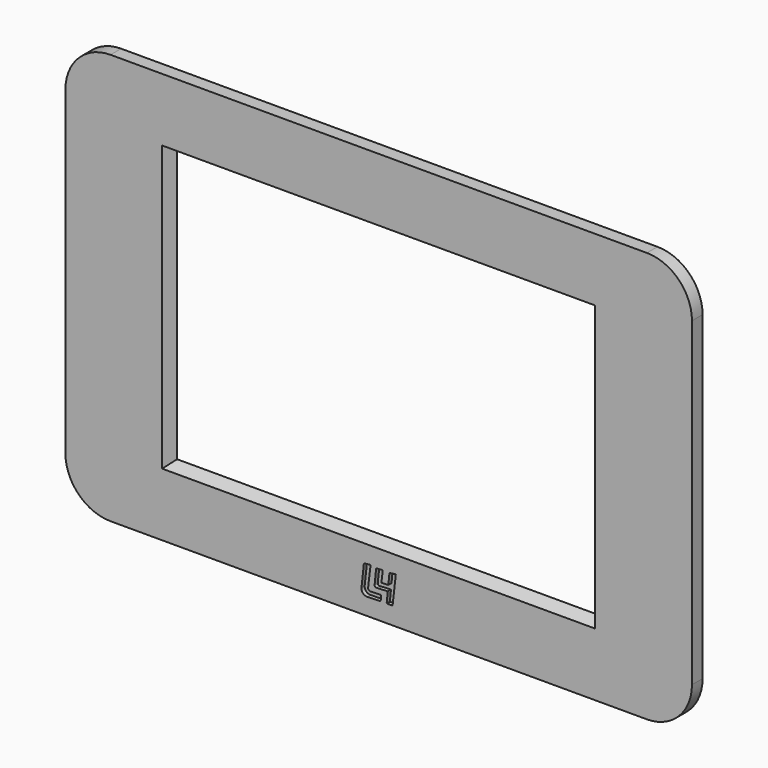
from build123d import *

# Parameters (mm, degrees)
F0_W     = 236.2
F0_H     = 154.8
F0_W_2   = 160
F0_H_2   = 104
F1_DEPTH = 5
F2_R     = 17
F3_R     = 3.25
F4_DEPTH = 2.5
F5_SIZE2 = 4.99999
F5_SIZE  = 1.624588
F7_DEPTH = 1.5


# Not quite as in the source:
# - a fillet or chamfer is up to 0.001 mm smaller than in the source, because OpenCascade refuses the exact size


with BuildPart() as f1:
    # F0 (on Front) → F1 (new body)
    with BuildSketch(Plane.XZ):
        Rectangle(F0_W, F0_H)
        Rectangle(F0_W_2, F0_H_2, mode=Mode.SUBTRACT)
    extrude(amount=F1_DEPTH)

    # F2
    f2_edges = [f1.edges().sort_by_distance(p)[0] for p in [
        (-118.1, -2.5, 77.4),
        (118.1, -2.5, 77.4),
        (-118.1, -2.5, -77.4),
        (118.1, -2.5, -77.4),
    ]]
    fillet(f2_edges, radius=F2_R)

    # F3 (on face) → F4 (cut)
    with BuildSketch(Plane(origin=(0, 0, 0), x_dir=(-1, 0, 0), z_dir=(0, 1, 0))):
        with Locations((-79.25, 66.42428)):
            Circle(F3_R)
        with Locations((-79.25, -66.42428)):
            Circle(F3_R)
        with Locations((79.25, 66.42428)):
            Circle(F3_R)
        with Locations((79.25, -66.42428)):
            Circle(F3_R)
    extrude(amount=-F4_DEPTH, mode=Mode.SUBTRACT)

    # F5 (size 1.6245984812 and 5 in the source; OpenCascade refuses exactly that, so slightly less here)
    f5_edges = [f1.edges().sort_by_distance(p)[0] for p in [
        (-80, -5, 0),
        (0, -5, 52),
        (80, -5, 0),
        (0, -5, -52),
    ]]
    f5_side = f1.faces().sort_by_distance((0, -5, 74.575934))[0]
    chamfer(f5_edges, length=F5_SIZE, length2=F5_SIZE2, reference=f5_side)

    # F6 (on face) → F7 (cut)
    with BuildSketch(Plane.XZ.offset(5)):
        with BuildLine():
            Line((0, -70.9037960887), (0, -68.7403732376))
            Line((0, -68.7403732376), (-3.125376912, -68.8479899255))
            ThreePointArc((-3.125376912, -68.8479899255), (-3.7805726372, -68.5735525412), (-3.998605605, -67.897491197))
            Line((-3.998605605, -67.897491197), (-3.0892937711, -60.2992490469))
            ThreePointArc((-3.0892937711, -60.2992490469), (-3.1618997395, -60.0916194181), (-3.3704565536, -60.021721316))
            Line((-3.3704565536, -60.021721316), (-5.3485393199, -60.2845971301))
            ThreePointArc((-5.3485393199, -60.2845971301), (-5.5237209211, -60.3724524554), (-5.6072790976, -60.5497239497))
            Line((-5.6072790976, -60.5497239497), (-6.4865739197, -68.6796104252))
            ThreePointArc((-6.4865739197, -68.6796104252), (-5.9450748854, -70.3262933271), (-4.3499759171, -71.004854352))
            Line((-4.3499759171, -71.004854352), (0, -70.9037960887))
        make_face()
        with BuildLine():
            Line((1.2918589674, -60.2652083751), (0, -60.3707235945))
            Line((0, -60.3707235945), (0, -66.8485857862))
            Line((0, -66.8485857862), (3.4268085146, -66.6858144104))
            Line((3.4268085146, -66.6858144104), (3.0311800837, -70.6349397286))
            ThreePointArc((3.0311800837, -70.6349397286), (3.0818813973, -70.7890639463), (3.2301839467, -70.8548761904))
            Line((3.2301839467, -70.8548761904), (5.0478271442, -70.8548761904))
            ThreePointArc((5.0478271442, -70.8548761904), (5.1809587177, -70.8041276029), (5.2465278981, -70.6776360316))
            Line((5.2465278981, -70.6776360316), (6.4378099563, -60.2773594464))
            ThreePointArc((6.4378099563, -60.2773594464), (6.3777706296, -60.1104711604), (6.2086864979, -60.0569269995))
            Line((6.2086864979, -60.0569269995), (4.2790884308, -60.3539008339))
            ThreePointArc((4.2790884308, -60.3539008339), (4.1073828743, -60.4436163854), (4.0263119894, -60.6195686231))
            Line((4.0263119894, -60.6195686231), (3.6252996651, -64.4996576011))
            Line((3.6252996651, -64.4996576011), (1.0174442614, -64.6235291889))
            Line((1.0174442614, -64.6235291889), (1.506754727, -60.4880446531))
            ThreePointArc((1.506754727, -60.4880446531), (1.4521032332, -60.3257114675), (1.2918589674, -60.2652083751))
        make_face()
        with BuildLine():
            Line((0, -66.8485857862), (0, -60.3707235945))
            Line((0, -60.3707235945), (-0.7053982188, -60.4283384346))
            ThreePointArc((-0.7053982188, -60.4283384346), (-0.8907958695, -60.512923053), (-0.9793808578, -60.6964429332))
            Line((-0.9793808578, -60.6964429332), (-1.552537239, -66.2315062229))
            ThreePointArc((-1.552537239, -66.2315062229), (-1.3916459971, -66.7055871007), (-0.9272608372, -66.892630127))
            Line((-0.9272608372, -66.892630127), (0, -66.8485857862))
        make_face()
        with BuildLine():
            Line((0.7437746725, -68.7147627052), (0, -68.7403732376))
            Line((0, -68.7403732376), (0, -70.9037960887))
            Line((0, -70.9037960887), (0.4531291197, -70.8932690322))
            ThreePointArc((0.4531291197, -70.8932690322), (0.6476972416, -70.8155735275), (0.7439755724, -70.6294987347))
            Line((0.7439755724, -70.6294987347), (0.9491999954, -68.9387434307))
            ThreePointArc((0.9491999954, -68.9387434307), (0.8980521088, -68.7794601123), (0.7437746725, -68.7147627052))
        make_face()
    extrude(amount=-F7_DEPTH, mode=Mode.SUBTRACT)


solid = f1.part
